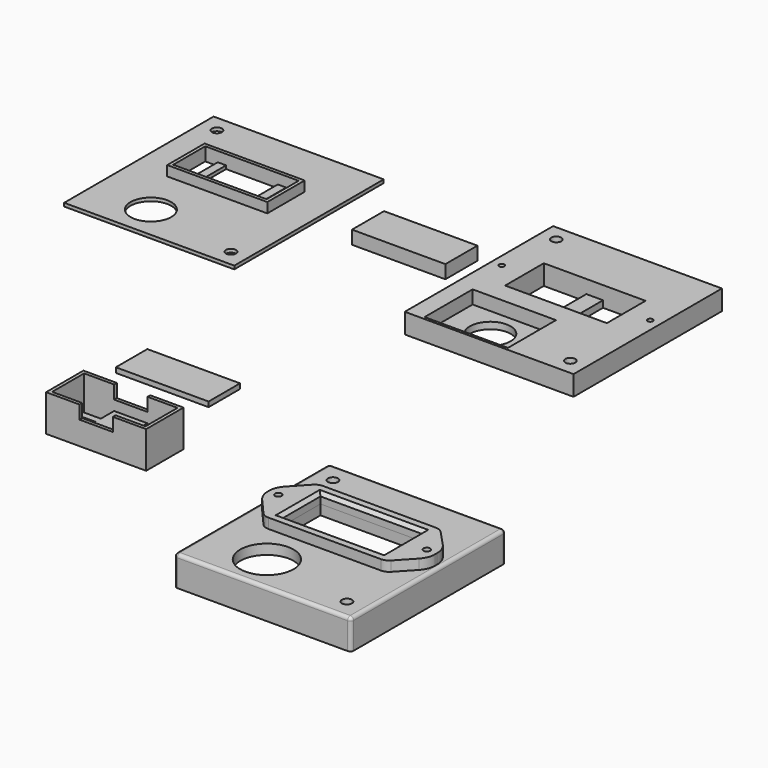
from build123d import *

# Parameters (mm, degrees)
F0_W      = 51
F0_H      = 56
F0_R      = 1.5
F0_R_2    = 6.1
F0_W_2    = 5
F0_H_2    = 14.5
F1_DEPTH  = 1
F0_W_3    = 2.5
F0_H_3    = 12
F3_W      = 28
F3_H      = 1
F4_DEPTH  = 3
F5_W      = 28
F5_H      = 12
F6_DEPTH  = 4
F7_T      = -1
F8_W      = 2
F8_H      = 10
F9_DEPTH  = 3
F2_W      = 30
F2_H      = 14
F11_DEPTH = 4
F2_W_2    = 51
F2_H_2    = 56
F2_R      = 8
F2_R_2    = 1.5
F2_R_3    = 0.8
F2_W_3    = 30.5
F2_H_3    = 14.5
F12_DEPTH = 3
F2_W_4    = 9
F2_H_4    = 2
F2_W_5    = 10
F2_H_5    = 5
F13_DEPTH = 1
F5_W_2    = 27.8
F5_H_2    = 11.8
F14_DEPTH = 1.5
F2_H_6    = 1
F15_DEPTH = 9
F16_W     = 36.5
F16_H     = 20.5
F16_W_2   = 30.5
F16_H_2   = 14.5
F16_R     = 1
F17_DEPTH = 3
F18_R     = 6
F19_R     = 3
F20_R     = 1
F21_SIZE  = 1
F23_W     = 9
F23_H     = 1
F24_DEPTH = 4
F25_DEPTH = 1
F26_D     = 1.4
F26_DEPTH = 1.001
F28_D     = 1.4
F27_W     = 1
F27_H     = 12
F29_DEPTH = 3
F22_W     = 51
F22_H     = 56
F22_W_2   = 25
F22_H_2   = 18
F22_R     = 1.5
F30_DEPTH = 5
F31_W     = 0.2
F31_H     = 55.6
F32_DEPTH = 25
F33_D     = 1.6
F33_DEPTH = 5.001
F34_D     = 1.6


# Not quite as in the source:
# - a feature names something its author has since deleted; it is built from what else it names


with BuildPart() as f1:
    # F0 (on Top) → F1 (new body)
    with BuildSketch(Plane.XY):
        Rectangle(F0_W, F0_H)
        with Locations((20.5, -23)):
            Circle(F0_R, mode=Mode.SUBTRACT)
        with Locations((-7.5, -18)):
            Circle(F0_R_2, mode=Mode.SUBTRACT)
        Polygon((-15.25, -2.75), (-15.25, 11.75), (-2.5, 11.75), (2.5, 11.75), (15.25, 11.75), (15.25, -2.75), (2.5, -2.75), (-2.5, -2.75), align=None, mode=Mode.SUBTRACT)
        with Locations((-20.5, 23)):
            Circle(F0_R, mode=Mode.SUBTRACT)
        with Locations((0, 4.5)):
            Rectangle(F0_W_2, F0_H_2)
    extrude(amount=F1_DEPTH)

    # F25 (add): a face of the model
    f25_faces = [f1.faces().sort_by_distance(p)[0] for p in [
        (0.3722548806, 0.1869472989, 1),
    ]]
    extrude(f25_faces, amount=F25_DEPTH)

    # F26 (through all, one way)
    with BuildSketch(Plane.XY.offset(1)):
        with Locations((-22.25, 4.75), (22.25, 4.75)):
            Circle(F26_D / 2)
    extrude(amount=-F26_DEPTH, mode=Mode.SUBTRACT)

    # F28 (through all)
    with Locations(Plane(origin=(0, 0, 1), x_dir=(1, 0, 0), z_dir=(0, 0, -1))):
        with Locations((-22.25, -4.75), (22.25, -4.75)):
            Hole(F28_D / 2)

    # F22 (on face) → F30 (join)
    with BuildSketch(Plane.XY.offset(1)):
        Rectangle(F22_W, F22_H)
        with Locations((-7.5, -18)):
            Rectangle(F22_W_2, F22_H_2, mode=Mode.SUBTRACT)
        with Locations((20.5, -23)):
            Circle(F22_R, mode=Mode.SUBTRACT)
        with Locations((-20.5, 23)):
            Circle(F22_R, mode=Mode.SUBTRACT)
        Polygon((-15.25, -2.75), (-15.25, 11.75), (-2.5, 11.75), (2.5, 11.75), (15.25, 11.75), (15.25, -2.75), (2.5, -2.75), (-2.5, -2.75), align=None, mode=Mode.SUBTRACT)
    extrude(amount=F30_DEPTH)

    # F31 (on face) → F32 (cut)
    with BuildSketch(Plane(origin=(0, 0, 0), x_dir=(1, 0, 0), z_dir=(0, 0, -1))):
        Polygon((25.5, 28), (-25.5, 28), (-25.5, 27.8), (-25.3, 27.8), (25.3, 27.8), (25.5, 27.8), align=None)
        with Locations((-25.4, 0)):
            Rectangle(F31_W, F31_H)
        with Locations((25.4, 0)):
            Rectangle(F31_W, F31_H)
        Polygon((-25.3, -27.8), (-25.5, -27.8), (-25.5, -28), (25.5, -28), (25.5, -27.8), (25.3, -27.8), align=None)
    extrude(amount=-F32_DEPTH, mode=Mode.SUBTRACT)

    # F33 (through all, one way)
    with BuildSketch(Plane(origin=(0, 0, 1), x_dir=(1, 0, 0), z_dir=(0, 0, -1))):
        with Locations((-22.25, -4.75), (22.25, -4.75)):
            Circle(F33_D / 2)
    extrude(amount=-F33_DEPTH, mode=Mode.SUBTRACT)

    # F34 (through all)
    with Locations(Plane.XY.offset(1)):
        with Locations((22.25, 4.75), (-22.25, 4.75)):
            Hole(F34_D / 2)


with BuildPart() as f1b:
    # F0 (on Top) → F1, piece 2 (new body)
    with BuildSketch(Plane.XY):
        with Locations((-102.5748546124, 1.0383715183)):
            Rectangle(F0_W, F0_H)
        with Locations((-110.0748546124, -16.9616284817)):
            Circle(F0_R_2, mode=Mode.SUBTRACT)
        with Locations((-82.0748546124, -21.9616284817)):
            Circle(F0_R, mode=Mode.SUBTRACT)
        Polygon((-116.5748546124, -0.4616284817), (-116.5748546124, 11.5383715183), (-112.8248546124, 11.5383715183), (-110.3248546124, 11.5383715183), (-94.8248546124, 11.5383715183), (-92.3248546124, 11.5383715183), (-88.5748546124, 11.5383715183), (-88.5748546124, -0.4616284817), (-92.3248546124, -0.4616284817), (-94.8248546124, -0.4616284817), (-110.3248546124, -0.4616284817), (-112.8248546124, -0.4616284817), align=None, mode=Mode.SUBTRACT)
        with Locations((-123.0748546124, 24.0383715183)):
            Circle(F0_R, mode=Mode.SUBTRACT)
        with Locations((-111.5748546124, 5.5383715183)):
            Rectangle(F0_W_3, F0_H_3)
        with Locations((-93.5748546124, 5.5383715183)):
            Rectangle(F0_W_3, F0_H_3)
    extrude(amount=F1_DEPTH)

    # F3 (on face) → F4 (join)
    with BuildSketch(Plane.XY.offset(1)):
        with Locations((-102.5748546124, 12.0383715183)):
            Rectangle(F3_W, F3_H)
        Polygon((-116.5748546124, -0.4616284817), (-116.5748546124, 11.5383715183), (-116.5748546124, 12.5383715183), (-117.5748546124, 12.5383715183), (-117.5748546124, -1.4616284817), (-116.5748546124, -1.4616284817), align=None)
        Polygon((-88.5748546124, 12.5383715183), (-88.5748546124, 11.5383715183), (-88.5748546124, -0.4616284817), (-88.5748546124, -1.4616284817), (-87.5748546124, -1.4616284817), (-87.5748546124, 12.5383715183), align=None)
        with Locations((-102.5748546124, -0.9616284817)):
            Rectangle(F3_W, F3_H)
    extrude(amount=F4_DEPTH)


with BuildPart() as f6:
    # F5 (on Top) → F6 (new body)
    with BuildSketch(Plane.XY):
        with Locations((-49.3556470275, 6)):
            Rectangle(F5_W, F5_H)
    extrude(amount=F6_DEPTH)

    # F7
    f7_openings = [f6.faces().sort_by_distance(p)[0] for p in [
        (-49.355647, 6, 0),
    ]]
    offset(amount=F7_T, openings=f7_openings)

    # F8 (on face) → F9 (join)
    with BuildSketch(Plane(origin=(0, 0, 3), x_dir=(1, 0, 0), z_dir=(0, 0, -1))):
        with Locations((-49.3556470275, -6)):
            Rectangle(F8_W, F8_H)
    extrude(amount=F9_DEPTH)


with BuildPart() as f11:
    # F2 (on Top) → F11 (new body)
    with BuildSketch(Plane.XY):
        with Locations((-48.0005137329, -108.0776734079)):
            Rectangle(F2_W, F2_H)
        Polygon((-62.0005137329, -107.0776734079), (-62.0005137329, -102.0776734079), (-53.0005137329, -102.0776734079), (-43.0005137329, -102.0776734079), (-34.0005137329, -102.0776734079), (-34.0005137329, -107.0776734079), (-34.0005137329, -109.0776734079), (-34.0005137329, -114.0776734079), (-43.0005137329, -114.0776734079), (-53.0005137329, -114.0776734079), (-62.0005137329, -114.0776734079), (-62.0005137329, -109.0776734079), align=None, mode=Mode.SUBTRACT)
    extrude(amount=F11_DEPTH)

    # F2 (on Top) → F13 (join)
    with BuildSketch(Plane.XY):
        with Locations((-57.5005137329, -108.0776734079)):
            Rectangle(F2_W_4, F2_H_4)
        with Locations((-48.0005137329, -108.0776734079)):
            Rectangle(F2_W_5, F2_H_4)
        with Locations((-38.5005137329, -108.0776734079)):
            Rectangle(F2_W_4, F2_H_4)
        with Locations((-48.0005137329, -104.5776734079)):
            Rectangle(F2_W_5, F2_H_5)
        with Locations((-48.0005137329, -111.5776734079)):
            Rectangle(F2_W_5, F2_H_5)
    extrude(amount=F13_DEPTH)

    # F23 (on face) → F24 (join)
    with BuildSketch(Plane.XY.offset(4)):
        Polygon((-53.0005137329, -101.0776734079), (-63.0005137329, -101.0776734079), (-63.0005137329, -102.0776734079), (-62.0005137329, -102.0776734079), (-53.0005137329, -102.0776734079), align=None)
        Polygon((-62.0005137329, -102.0776734079), (-63.0005137329, -102.0776734079), (-63.0005137329, -115.0776734079), (-62.0005137329, -115.0776734079), (-62.0005137329, -114.0776734079), align=None)
        with Locations((-57.5005137329, -114.5776734079)):
            Rectangle(F23_W, F23_H)
        Polygon((-33.0005137329, -102.0776734079), (-33.0005137329, -101.0776734079), (-43.0005137329, -101.0776734079), (-43.0005137329, -102.0776734079), (-34.0005137329, -102.0776734079), align=None)
        Polygon((-33.0005137329, -115.0776734079), (-33.0005137329, -102.0776734079), (-34.0005137329, -102.0776734079), (-34.0005137329, -114.0776734079), (-34.0005137329, -115.0776734079), align=None)
        with Locations((-38.5005137329, -114.5776734079)):
            Rectangle(F23_W, F23_H)
    extrude(amount=F24_DEPTH)

    # F27 (on face) → F29 (join)
    with BuildSketch(Plane(origin=(0, 0, 0), x_dir=(1, 0, 0), z_dir=(0, 0, -1))):
        Polygon((-33.0005137329, 115.0776734079), (-63.0005137329, 115.0776734079), (-63.0005137329, 114.0776734079), (-62.0005137329, 114.0776734079), (-34.0005137329, 114.0776734079), (-33.0005137329, 114.0776734079), align=None)
        Polygon((-62.0005137329, 114.0776734079), (-63.0005137329, 114.0776734079), (-63.0005137329, 101.0776734079), (-62.0005137329, 101.0776734079), (-62.0005137329, 102.0776734079), align=None)
        with Locations((-33.5005137329, 108.0776734079)):
            Rectangle(F27_W, F27_H)
        Polygon((-33.0005137329, 101.0776734079), (-33.0005137329, 102.0776734079), (-34.0005137329, 102.0776734079), (-62.0005137329, 102.0776734079), (-62.0005137329, 101.0776734079), align=None)
    extrude(amount=F29_DEPTH)


with BuildPart() as f12:
    # F2 (on Top) → F12 (new body)
    with BuildSketch(Plane.XY):
        with Locations((28.2103444552, -118.9687541723)):
            Rectangle(F2_W_2, F2_H_2)
        with Locations((20.7103444552, -136.9687541723)):
            Circle(F2_R, mode=Mode.SUBTRACT)
        with Locations((48.7103444552, -141.9687541723)):
            Circle(F2_R_2, mode=Mode.SUBTRACT)
        with Locations((5.9603444552, -114.2187541723)):
            Circle(F2_R_3, mode=Mode.SUBTRACT)
        with Locations((28.2103444552, -114.4687541723)):
            Rectangle(F2_W_3, F2_H_3, mode=Mode.SUBTRACT)
        with Locations((50.4603444552, -114.2187541723)):
            Circle(F2_R_3, mode=Mode.SUBTRACT)
        with Locations((7.7103444552, -95.9687541723)):
            Circle(F2_R_2, mode=Mode.SUBTRACT)
    extrude(amount=-F12_DEPTH)

    # F2 (on Top) → F15 (join)
    with BuildSketch(Plane.XY):
        Polygon((2.7103444552, -146.9687541723), (2.7103444552, -90.9687541723), (2.7103444552, -89.9687541723), (1.7103444552, -89.9687541723), (1.7103444552, -147.9687541723), (2.7103444552, -147.9687541723), align=None)
        with Locations((28.2103444552, -90.4687541723)):
            Rectangle(F2_W_2, F2_H_6)
        with Locations((28.2103444552, -147.4687541723)):
            Rectangle(F2_W_2, F2_H_6)
        Polygon((53.7103444552, -89.9687541723), (53.7103444552, -90.9687541723), (53.7103444552, -146.9687541723), (53.7103444552, -147.9687541723), (54.7103444552, -147.9687541723), (54.7103444552, -89.9687541723), align=None)
    extrude(amount=-F15_DEPTH)

    # F20
    f20_edges = [f12.edges().sort_by_distance(p)[0] for p in [
        (1.710344, -118.968754, 0),
        (28.210344, -89.968754, 0),
        (28.210344, -147.968754, 0),
        (54.710344, -118.968754, 0),
        (54.710344, -147.968754, -4.5),
        (1.710344, -147.968754, -4.5),
        (1.710344, -89.968754, -4.5),
        (54.710344, -89.968754, -4.5),
    ]]
    fillet(f20_edges, radius=F20_R)


with BuildPart() as f14:
    # F5 (on Top) → F14 (new body)
    with BuildSketch(Plane.XY):
        with Locations((-52.0366017878, -79.3675661445)):
            Rectangle(F5_W_2, F5_H_2)
    extrude(amount=F14_DEPTH)


with BuildPart() as f17:
    # F16 (on face) → F17 (new body)
    with BuildSketch(Plane.XY):
        with Locations((28.2103444552, -114.4687541723)):
            Rectangle(F16_W, F16_H)
        with Locations((28.2103444552, -114.4687541723)):
            Rectangle(F16_W_2, F16_H_2, mode=Mode.SUBTRACT)
        Polygon((9.9603444552, -124.7187541723), (9.9603444552, -104.2187541723), (2.9603444552, -111.7187541723), (2.9603444552, -116.7187541723), align=None)
        with Locations((5.9603444552, -114.2187541723)):
            Circle(F16_R, mode=Mode.SUBTRACT)
        Polygon((53.4603444552, -111.7187541723), (46.4603444552, -104.2187541723), (46.4603444552, -124.7187541723), (53.4603444552, -117.2187541723), align=None)
        with Locations((50.4603444552, -114.2187541723)):
            Circle(F16_R, mode=Mode.SUBTRACT)
    extrude(amount=F17_DEPTH)

    # F18
    f18_edges = [f17.edges().sort_by_distance(p)[0] for p in [
        (2.960344, -111.718754, 1.5),
        (2.960344, -116.718754, 1.5),
        (53.460344, -117.218754, 1.5),
        (53.460344, -111.718754, 1.5),
    ]]
    fillet(f18_edges, radius=F18_R)

    # F19
    f19_edges = [f17.edges().sort_by_distance(p)[0] for p in [
        (9.960344, -104.218754, 1.5),
        (9.960344, -124.718754, 1.5),
        (46.460344, -124.718754, 1.5),
        (46.460344, -104.218754, 1.5),
    ]]
    fillet(f19_edges, radius=F19_R)

    # F21
    f21_edges = [f17.edges().sort_by_distance(p)[0] for p in [
        (12.960344, -114.468754, 3),
        (28.210344, -107.218754, 3),
        (43.460344, -114.468754, 3),
        (28.210344, -121.718754, 3),
    ]]
    chamfer(f21_edges, length=F21_SIZE)


solid = Compound([f1.part, f1b.part, f6.part, f11.part, f12.part, f14.part, f17.part])
